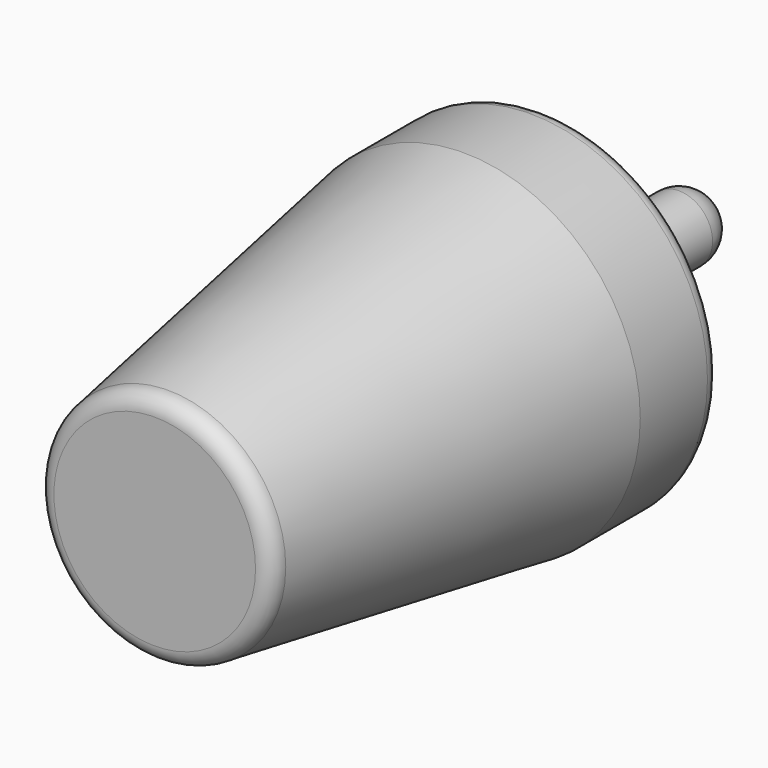
from build123d import *

# Parameters (mm, degrees)
F2_R      = 3.5
F3_DEPTH  = 0.5
F0_R      = 5.25
F4_DEPTH  = 3
F5_R      = 1
F6_DEPTH  = 6
F3_FACE_R = 3.5
F4_FACE_R = 5.25
F8_R      = 0.49999
F9_R      = 0.5
F10_R     = 1


# Not quite as in the source:
# - a fillet or chamfer is up to 0.001 mm smaller than in the source, because OpenCascade refuses the exact size


with BuildPart() as f3:
    # F2 (on offset) → F3 (new body)
    with BuildSketch(Plane.XZ.offset(14)):
        Circle(F2_R)
    extrude(amount=F3_DEPTH)

    # F8 (radius 0.5 in the source; OpenCascade refuses exactly that, so slightly less here)
    f8_edges = [f3.edges().sort_by_distance(p)[0] for p in [
        (-3.5, -14.5, 0),
    ]]
    fillet(f8_edges, radius=F8_R)


with BuildPart() as f4:
    # F0 (on Front) → F4 (new body)
    with BuildSketch(Plane.XZ):
        Circle(F0_R)
    extrude(amount=F4_DEPTH)

    # F5 (on Front) → F6 (join)
    with BuildSketch(Plane.XZ):
        Circle(F5_R)
    extrude(amount=-F6_DEPTH)

    # F9
    f9_edges = [f4.edges().sort_by_distance(p)[0] for p in [
        (-5.25, 0, 0),
    ]]
    fillet(f9_edges, radius=F9_R)

    # F10
    f10_edges = [f4.edges().sort_by_distance(p)[0] for p in [
        (-1, 6, 0),
    ]]
    fillet(f10_edges, radius=F10_R)


with BuildPart() as f7:
    # F3_face (on face) → F7 section 0
    with BuildSketch(Plane(origin=(0, -14, 0), x_dir=(1, 0, 0), z_dir=(0, 1, 0))):
        Circle(F3_FACE_R)
    # F4_face (on face) → F7 section 1
    with BuildSketch(Plane.XZ.offset(3)):
        Circle(F4_FACE_R)
    loft()


solid = Compound([f3.part, f4.part, f7.part])
